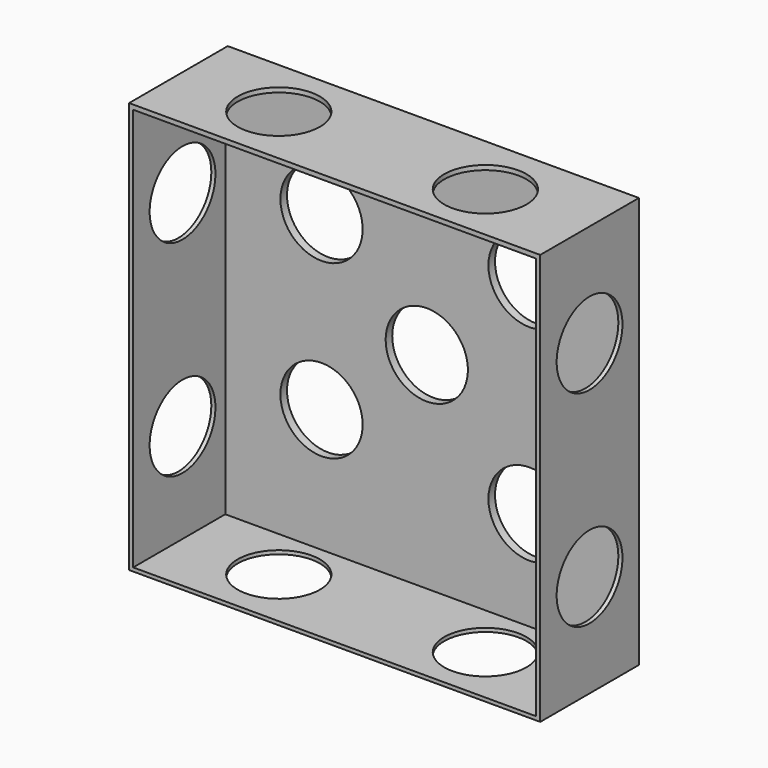
from build123d import *

# Parameters (mm, degrees)
F0_W     = 100
F0_H     = 100
F1_DEPTH = 30
F2_R     = 10
F3_DEPTH = 100
F4_R     = 10
F5_DEPTH = 100
F6_W     = 98
F6_H     = 98
F7_DEPTH = 28
F8_R     = 10
F9_DEPTH = 3


# Not quite as in the source:
# - a feature names something its author has since deleted; it is built from what else it names


with BuildPart() as f1:
    # F0 (on Front) → F1 (new body)
    with BuildSketch(Plane.XZ):
        with Locations((25.5921050906, -0.9599315155)):
            Rectangle(F0_W, F0_H)
    extrude(amount=-F1_DEPTH)

    # F2 (on face) → F3 (cut)
    with BuildSketch(Plane.YZ.offset(75.5921050906)):
        with Locations((15, 24.0400684845)):
            Circle(F2_R)
        with Locations((15, -25.9599315155)):
            Circle(F2_R)
    extrude(amount=-F3_DEPTH, mode=Mode.SUBTRACT)

    # F4 (on face) → F5 (cut)
    with BuildSketch(Plane.XY.offset(49.0400684845)):
        with Locations((0, 15)):
            Circle(F4_R)
        with Locations((50.5921050906, 14.5671376958)):
            Circle(F4_R)
    extrude(amount=-F5_DEPTH, mode=Mode.SUBTRACT)

    # F6 (on face) → F7 (cut)
    with BuildSketch(Plane.XZ):
        with Locations((25.5921050906, -1.0704044253)):
            Rectangle(F6_W, F6_H)
    extrude(amount=-F7_DEPTH, mode=Mode.SUBTRACT)

    # F8 (on face) → F9 (cut)
    with BuildSketch(Plane(origin=(0, 30, 0), x_dir=(-1, 0, 0), z_dir=(0, 1, 0))):
        with Locations((0, -20.037606527)):
            Circle(F8_R)
        with Locations((0, 21.7908981225)):
            Circle(F8_R)
        with Locations((-25.5921050906, 0)):
            Circle(F8_R)
        with Locations((-50.5921050906, 24.0400684845)):
            Circle(F8_R)
        with Locations((-50.5921050906, -25.9599315155)):
            Circle(F8_R)
    extrude(amount=-F9_DEPTH, mode=Mode.SUBTRACT)


solid = f1.part
